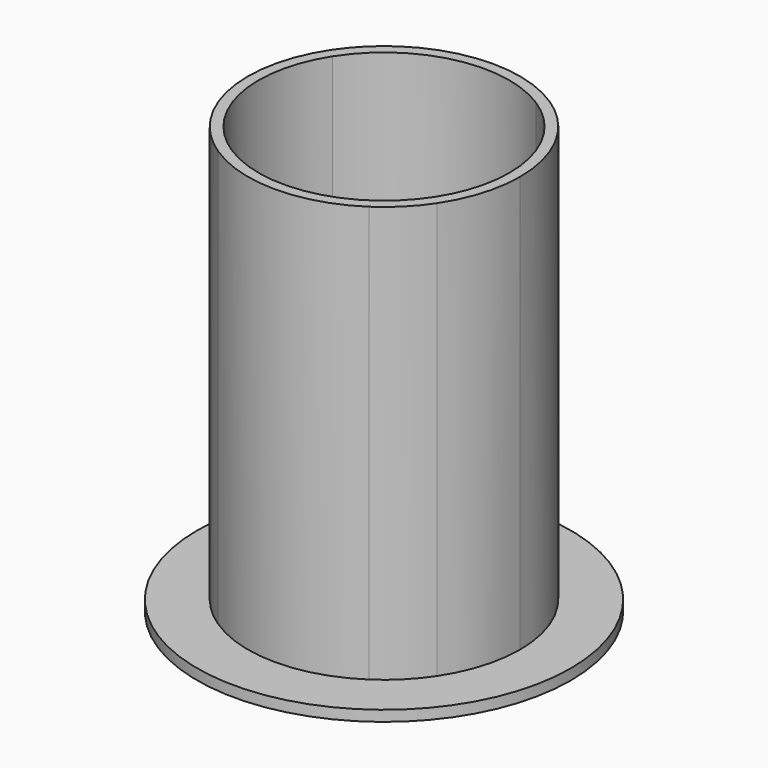
from build123d import *

# Parameters (mm, degrees)
F0_R     = 35
F0_R_2   = 2.4
F1_DEPTH = 2
F2_DEPTH = 80
F3_DEPTH = 5.5


# Not quite as in the source:
# - a feature names something its author has since deleted; it is built from what else it names


with BuildPart() as f1:
    # F0 (on Top) → F1 (new body)
    with BuildSketch(Plane.XY):
        with Locations((-1.1396982046, 1.6525272475)):
            Circle(F0_R)
        with BuildLine():
            ThreePointArc((24.3603017954, 1.6525272475), (23.2660064022, -5.7374377488), (20.0770404114, -12.4931435567))
            ThreePointArc((20.0770404114, -12.4931435567), (16.8915247156, -16.3786956728), (13.0059725995, -19.5642113686))
            ThreePointArc((13.0059725995, -19.5642113686), (-1.1396982046, -23.8474727525), (-15.2853690088, -19.5642113686))
            ThreePointArc((-15.2853690088, -19.5642113686), (-19.1709211249, -16.3786956728), (-22.3564368206, -12.4931435567))
            ThreePointArc((-22.3564368206, -12.4931435567), (-26.6396982046, 1.6525272475), (-22.3564368206, 15.7981980516))
            ThreePointArc((-22.3564368206, 15.7981980516), (-19.1709211249, 19.6837501677), (-15.2853690088, 22.8692658635))
            ThreePointArc((-15.2853690088, 22.8692658635), (-1.1396982046, 27.1525272475), (13.0059725995, 22.8692658635))
            ThreePointArc((13.0059725995, 22.8692658635), (16.8915247156, 19.6837501677), (20.0770404114, 15.7981980516))
            ThreePointArc((20.0770404114, 15.7981980516), (23.2660064022, 9.0424922437), (24.3603017954, 1.6525272475))
        make_face(mode=Mode.SUBTRACT)
        with BuildLine():
            ThreePointArc((11.5613007706, -18.1195395396), (15.4773111533, -14.9644821104), (18.6323685824, -11.0484717277))
            ThreePointArc((18.6323685824, -11.0484717277), (21.4090663901, -4.9658725026), (22.3603017954, 1.6525272475))
            ThreePointArc((22.3603017954, 1.6525272475), (21.4090663901, 8.2709269976), (18.6323685824, 14.3535262227))
            ThreePointArc((18.6323685824, 14.3535262227), (15.4773111533, 18.2695366053), (11.5613007706, 21.4245940345))
            ThreePointArc((11.5613007706, 21.4245940345), (-1.1396982046, 25.1525272475), (-13.8406971798, 21.4245940345))
            ThreePointArc((-13.8406971798, 21.4245940345), (-17.7567075625, 18.2695366053), (-20.9117649917, 14.3535262227))
            ThreePointArc((-20.9117649917, 14.3535262227), (-24.6396982046, 1.6525272475), (-20.9117649917, -11.0484717277))
            ThreePointArc((-20.9117649917, -11.0484717277), (-17.7567075625, -14.9644821104), (-13.8406971798, -18.1195395396))
            ThreePointArc((-13.8406971798, -18.1195395396), (-1.1396982046, -21.8474727525), (11.5613007706, -18.1195395396))
        make_face()
        Polygon((1.7603017954, -5.5474727525), (1.7603017954, -7.5474727525), (-4.0396982046, -7.5474727525), (-4.0396982046, -5.5474727525), (-6.0396982046, -5.5474727525), (-6.0396982046, -4.5474727525), (-3.6396982046, -2.7474727525), (1.3603017954, -2.7474727525), (3.7603017954, -4.5474727525), (3.7603017954, -5.5474727525), align=None, mode=Mode.SUBTRACT)
        Polygon((-8.3396982046, -1.2474727525), (-10.3396982046, -1.2474727525), (-10.3396982046, 4.5525272475), (-8.3396982046, 4.5525272475), (-8.3396982046, 6.5525272475), (-7.3396982046, 6.5525272475), (-5.5396982046, 4.1525272475), (-5.5396982046, -0.8474727525), (-7.3396982046, -3.2474727525), (-8.3396982046, -3.2474727525), align=None, mode=Mode.SUBTRACT)
        Polygon((1.7603017954, 8.8525272475), (3.7603017954, 8.8525272475), (3.7603017954, 7.8525272475), (1.3603017954, 6.0525272475), (-3.6396982046, 6.0525272475), (-6.0396982046, 7.8525272475), (-6.0396982046, 8.8525272475), (-4.0396982046, 8.8525272475), (-4.0396982046, 10.8525272475), (1.7603017954, 10.8525272475), align=None, mode=Mode.SUBTRACT)
        with Locations((-1.1396982046, 1.6525272475)):
            Circle(F0_R_2, mode=Mode.SUBTRACT)
        Polygon((5.0603017954, -3.2474727525), (3.2603017954, -0.8474727525), (3.2603017954, 4.1525272475), (5.0603017954, 6.5525272475), (6.0603017954, 6.5525272475), (6.0603017954, 4.5525272475), (8.0603017954, 4.5525272475), (8.0603017954, -1.2474727525), (6.0603017954, -1.2474727525), (6.0603017954, -3.2474727525), align=None, mode=Mode.SUBTRACT)
        with BuildLine():
            Line((18.6323685824, -11.0484717277), (20.0770404114, -12.4931435567))
            ThreePointArc((20.0770404114, -12.4931435567), (23.2660064022, -5.7374377488), (24.3603017954, 1.6525272475))
            ThreePointArc((24.3603017954, 1.6525272475), (23.2660064022, 9.0424922437), (20.0770404114, 15.7981980516))
            Line((20.0770404114, 15.7981980516), (18.6323685824, 14.3535262227))
            ThreePointArc((18.6323685824, 14.3535262227), (21.4090663901, 8.2709269976), (22.3603017954, 1.6525272475))
            ThreePointArc((22.3603017954, 1.6525272475), (21.4090663901, -4.9658725026), (18.6323685824, -11.0484717277))
        make_face()
        with BuildLine():
            ThreePointArc((-15.2853690088, -19.5642113686), (-1.1396982046, -23.8474727525), (13.0059725995, -19.5642113686))
            Line((13.0059725995, -19.5642113686), (11.5613007706, -18.1195395396))
            ThreePointArc((11.5613007706, -18.1195395396), (-1.1396982046, -21.8474727525), (-13.8406971798, -18.1195395396))
            Line((-13.8406971798, -18.1195395396), (-15.2853690088, -19.5642113686))
        make_face()
        with BuildLine():
            Line((11.5613007706, 21.4245940345), (13.0059725995, 22.8692658635))
            ThreePointArc((13.0059725995, 22.8692658635), (-1.1396982046, 27.1525272475), (-15.2853690088, 22.8692658635))
            Line((-15.2853690088, 22.8692658635), (-13.8406971798, 21.4245940345))
            ThreePointArc((-13.8406971798, 21.4245940345), (-1.1396982046, 25.1525272475), (11.5613007706, 21.4245940345))
        make_face()
        with BuildLine():
            ThreePointArc((-22.3564368206, 15.7981980516), (-26.6396982046, 1.6525272475), (-22.3564368206, -12.4931435567))
            Line((-22.3564368206, -12.4931435567), (-20.9117649917, -11.0484717277))
            ThreePointArc((-20.9117649917, -11.0484717277), (-24.6396982046, 1.6525272475), (-20.9117649917, 14.3535262227))
            Line((-20.9117649917, 14.3535262227), (-22.3564368206, 15.7981980516))
        make_face()
        Polygon((-10.3396982046, 4.5525272475), (-10.3396982046, -1.2474727525), (-8.3396982046, -1.2474727525), (-8.3396982046, -3.2474727525), (-7.3396982046, -3.2474727525), (-5.5396982046, -0.8474727525), (-5.5396982046, 4.1525272475), (-7.3396982046, 6.5525272475), (-8.3396982046, 6.5525272475), (-8.3396982046, 4.5525272475), align=None)
        Polygon((3.2603017954, 4.1525272475), (3.2603017954, -0.8474727525), (5.0603017954, -3.2474727525), (6.0603017954, -3.2474727525), (6.0603017954, -1.2474727525), (8.0603017954, -1.2474727525), (8.0603017954, 4.5525272475), (6.0603017954, 4.5525272475), (6.0603017954, 6.5525272475), (5.0603017954, 6.5525272475), align=None)
        Polygon((-4.0396982046, -7.5474727525), (1.7603017954, -7.5474727525), (1.7603017954, -5.5474727525), (3.7603017954, -5.5474727525), (3.7603017954, -4.5474727525), (1.3603017954, -2.7474727525), (-3.6396982046, -2.7474727525), (-6.0396982046, -4.5474727525), (-6.0396982046, -5.5474727525), (-4.0396982046, -5.5474727525), align=None)
        Polygon((3.7603017954, 7.8525272475), (3.7603017954, 8.8525272475), (1.7603017954, 8.8525272475), (1.7603017954, 10.8525272475), (-4.0396982046, 10.8525272475), (-4.0396982046, 8.8525272475), (-6.0396982046, 8.8525272475), (-6.0396982046, 7.8525272475), (-3.6396982046, 6.0525272475), (1.3603017954, 6.0525272475), align=None)
        with BuildLine():
            ThreePointArc((13.0059725995, -19.5642113686), (16.8915247156, -16.3786956728), (20.0770404114, -12.4931435567))
            Line((20.0770404114, -12.4931435567), (18.6323685824, -11.0484717277))
            ThreePointArc((18.6323685824, -11.0484717277), (15.4773111533, -14.9644821104), (11.5613007706, -18.1195395396))
            Line((11.5613007706, -18.1195395396), (13.0059725995, -19.5642113686))
        make_face()
        with BuildLine():
            Line((18.6323685824, 14.3535262227), (20.0770404114, 15.7981980516))
            ThreePointArc((20.0770404114, 15.7981980516), (16.8915247156, 19.6837501677), (13.0059725995, 22.8692658635))
            Line((13.0059725995, 22.8692658635), (11.5613007706, 21.4245940345))
            ThreePointArc((11.5613007706, 21.4245940345), (15.4773111533, 18.2695366053), (18.6323685824, 14.3535262227))
        make_face()
        with BuildLine():
            ThreePointArc((-22.3564368206, -12.4931435567), (-19.1709211249, -16.3786956728), (-15.2853690088, -19.5642113686))
            Line((-15.2853690088, -19.5642113686), (-13.8406971798, -18.1195395396))
            ThreePointArc((-13.8406971798, -18.1195395396), (-17.7567075625, -14.9644821104), (-20.9117649917, -11.0484717277))
            Line((-20.9117649917, -11.0484717277), (-22.3564368206, -12.4931435567))
        make_face()
        with BuildLine():
            Line((-13.8406971798, 21.4245940345), (-15.2853690088, 22.8692658635))
            ThreePointArc((-15.2853690088, 22.8692658635), (-19.1709211249, 19.6837501677), (-22.3564368206, 15.7981980516))
            Line((-22.3564368206, 15.7981980516), (-20.9117649917, 14.3535262227))
            ThreePointArc((-20.9117649917, 14.3535262227), (-17.7567075625, 18.2695366053), (-13.8406971798, 21.4245940345))
        make_face()
        with Locations((-1.1396982046, 1.6525272475)):
            Circle(F0_R_2)
    extrude(amount=F1_DEPTH)

    # F0 (on Top) → F2 (join)
    with BuildSketch(Plane.XY):
        with BuildLine():
            Line((11.5613007706, 21.4245940345), (13.0059725995, 22.8692658635))
            ThreePointArc((13.0059725995, 22.8692658635), (-1.1396982046, 27.1525272475), (-15.2853690088, 22.8692658635))
            Line((-15.2853690088, 22.8692658635), (-13.8406971798, 21.4245940345))
            ThreePointArc((-13.8406971798, 21.4245940345), (-1.1396982046, 25.1525272475), (11.5613007706, 21.4245940345))
        make_face()
        with BuildLine():
            ThreePointArc((-22.3564368206, 15.7981980516), (-26.6396982046, 1.6525272475), (-22.3564368206, -12.4931435567))
            Line((-22.3564368206, -12.4931435567), (-20.9117649917, -11.0484717277))
            ThreePointArc((-20.9117649917, -11.0484717277), (-24.6396982046, 1.6525272475), (-20.9117649917, 14.3535262227))
            Line((-20.9117649917, 14.3535262227), (-22.3564368206, 15.7981980516))
        make_face()
        with BuildLine():
            ThreePointArc((-15.2853690088, -19.5642113686), (-1.1396982046, -23.8474727525), (13.0059725995, -19.5642113686))
            Line((13.0059725995, -19.5642113686), (11.5613007706, -18.1195395396))
            ThreePointArc((11.5613007706, -18.1195395396), (-1.1396982046, -21.8474727525), (-13.8406971798, -18.1195395396))
            Line((-13.8406971798, -18.1195395396), (-15.2853690088, -19.5642113686))
        make_face()
        with BuildLine():
            Line((18.6323685824, -11.0484717277), (20.0770404114, -12.4931435567))
            ThreePointArc((20.0770404114, -12.4931435567), (23.2660064022, -5.7374377488), (24.3603017954, 1.6525272475))
            ThreePointArc((24.3603017954, 1.6525272475), (23.2660064022, 9.0424922437), (20.0770404114, 15.7981980516))
            Line((20.0770404114, 15.7981980516), (18.6323685824, 14.3535262227))
            ThreePointArc((18.6323685824, 14.3535262227), (21.4090663901, 8.2709269976), (22.3603017954, 1.6525272475))
            ThreePointArc((22.3603017954, 1.6525272475), (21.4090663901, -4.9658725026), (18.6323685824, -11.0484717277))
        make_face()
        with BuildLine():
            ThreePointArc((13.0059725995, -19.5642113686), (16.8915247156, -16.3786956728), (20.0770404114, -12.4931435567))
            Line((20.0770404114, -12.4931435567), (18.6323685824, -11.0484717277))
            ThreePointArc((18.6323685824, -11.0484717277), (15.4773111533, -14.9644821104), (11.5613007706, -18.1195395396))
            Line((11.5613007706, -18.1195395396), (13.0059725995, -19.5642113686))
        make_face()
        with BuildLine():
            Line((18.6323685824, 14.3535262227), (20.0770404114, 15.7981980516))
            ThreePointArc((20.0770404114, 15.7981980516), (16.8915247156, 19.6837501677), (13.0059725995, 22.8692658635))
            Line((13.0059725995, 22.8692658635), (11.5613007706, 21.4245940345))
            ThreePointArc((11.5613007706, 21.4245940345), (15.4773111533, 18.2695366053), (18.6323685824, 14.3535262227))
        make_face()
        with BuildLine():
            Line((-13.8406971798, 21.4245940345), (-15.2853690088, 22.8692658635))
            ThreePointArc((-15.2853690088, 22.8692658635), (-19.1709211249, 19.6837501677), (-22.3564368206, 15.7981980516))
            Line((-22.3564368206, 15.7981980516), (-20.9117649917, 14.3535262227))
            ThreePointArc((-20.9117649917, 14.3535262227), (-17.7567075625, 18.2695366053), (-13.8406971798, 21.4245940345))
        make_face()
        with BuildLine():
            ThreePointArc((-22.3564368206, -12.4931435567), (-19.1709211249, -16.3786956728), (-15.2853690088, -19.5642113686))
            Line((-15.2853690088, -19.5642113686), (-13.8406971798, -18.1195395396))
            ThreePointArc((-13.8406971798, -18.1195395396), (-17.7567075625, -14.9644821104), (-20.9117649917, -11.0484717277))
            Line((-20.9117649917, -11.0484717277), (-22.3564368206, -12.4931435567))
        make_face()
    extrude(amount=F2_DEPTH)

    # F0 (on Top) → F3 (join)
    with BuildSketch(Plane.XY):
        Polygon((-10.3396982046, 4.5525272475), (-10.3396982046, -1.2474727525), (-8.3396982046, -1.2474727525), (-8.3396982046, -3.2474727525), (-7.3396982046, -3.2474727525), (-5.5396982046, -0.8474727525), (-5.5396982046, 4.1525272475), (-7.3396982046, 6.5525272475), (-8.3396982046, 6.5525272475), (-8.3396982046, 4.5525272475), align=None)
        Polygon((3.2603017954, 4.1525272475), (3.2603017954, -0.8474727525), (5.0603017954, -3.2474727525), (6.0603017954, -3.2474727525), (6.0603017954, -1.2474727525), (8.0603017954, -1.2474727525), (8.0603017954, 4.5525272475), (6.0603017954, 4.5525272475), (6.0603017954, 6.5525272475), (5.0603017954, 6.5525272475), align=None)
        Polygon((-4.0396982046, -7.5474727525), (1.7603017954, -7.5474727525), (1.7603017954, -5.5474727525), (3.7603017954, -5.5474727525), (3.7603017954, -4.5474727525), (1.3603017954, -2.7474727525), (-3.6396982046, -2.7474727525), (-6.0396982046, -4.5474727525), (-6.0396982046, -5.5474727525), (-4.0396982046, -5.5474727525), align=None)
        Polygon((3.7603017954, 7.8525272475), (3.7603017954, 8.8525272475), (1.7603017954, 8.8525272475), (1.7603017954, 10.8525272475), (-4.0396982046, 10.8525272475), (-4.0396982046, 8.8525272475), (-6.0396982046, 8.8525272475), (-6.0396982046, 7.8525272475), (-3.6396982046, 6.0525272475), (1.3603017954, 6.0525272475), align=None)
        with Locations((-1.1396982046, 1.6525272475)):
            Circle(F0_R_2)
    extrude(amount=-F3_DEPTH)


solid = f1.part
